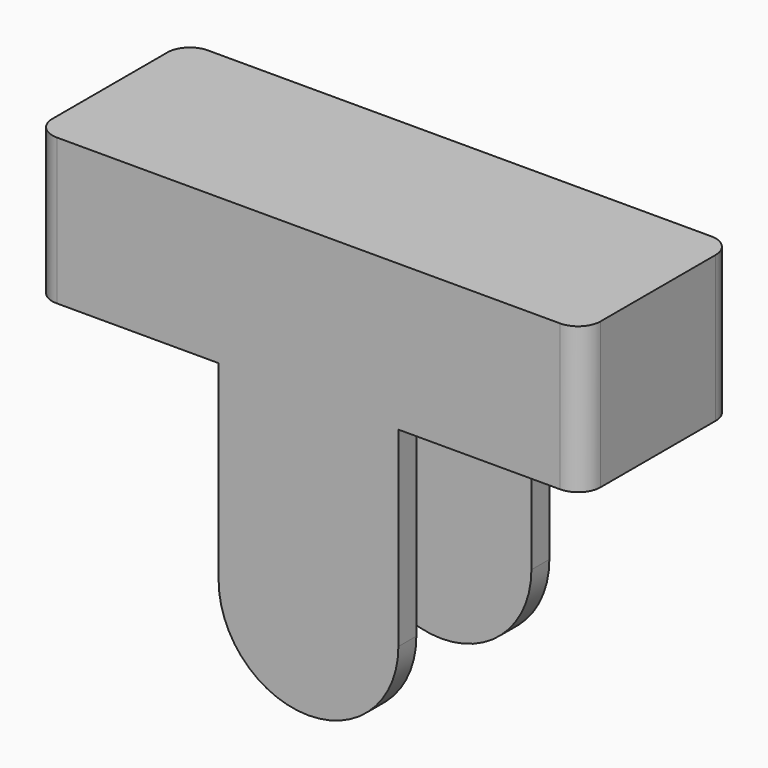
from build123d import *

# Parameters (mm, degrees)
F0_W     = 48.799998641
F0_H     = 16.799998641
F0_W_2   = 44.799998641
F0_H_2   = 12.799998641
F0_W_3   = 44
F0_H_3   = 12
F0_W_4   = 40
F0_H_4   = 8
F1_DEPTH = 13
F2_DEPTH = 10.5
F3_R     = 2
F4_R     = 2
F6_DEPTH = 25
F7_R     = 7.99999


# Not quite as in the source:
# - a fillet or chamfer is up to 0.001 mm smaller than in the source, because OpenCascade refuses the exact size


with BuildPart() as f1:
    # F0 (on Top) → F1 (new body)
    with BuildSketch(Plane.XY):
        Rectangle(F0_W, F0_H)
        Rectangle(F0_W_2, F0_H_2, mode=Mode.SUBTRACT)
        Rectangle(F0_W_2, F0_H_2)
        Rectangle(F0_W_3, F0_H_3, mode=Mode.SUBTRACT)
        Rectangle(F0_W_3, F0_H_3)
        Rectangle(F0_W_4, F0_H_4, mode=Mode.SUBTRACT)
        Rectangle(F0_W_4, F0_H_4)
    extrude(amount=F1_DEPTH)

    # F0 (on Top) → F2 (cut)
    with BuildSketch(Plane.XY):
        Rectangle(F0_W_2, F0_H_2)
        Rectangle(F0_W_3, F0_H_3, mode=Mode.SUBTRACT)
        Rectangle(F0_W_3, F0_H_3)
        Rectangle(F0_W_4, F0_H_4, mode=Mode.SUBTRACT)
        Rectangle(F0_W_4, F0_H_4)
    extrude(amount=F2_DEPTH, mode=Mode.SUBTRACT)

    # F3
    f3_edges = [f1.edges().sort_by_distance(p)[0] for p in [
        (-24.399999, -8.399999, 6.5),
        (-24.399999, 8.399999, 6.5),
        (24.399999, -8.399999, 6.5),
        (24.399999, 8.399999, 6.5),
    ]]
    fillet(f3_edges, radius=F3_R)

    # F4
    f4_edges = [f1.edges().sort_by_distance(p)[0] for p in [
        (-22.399999, -6.399999, 5.25),
        (22.399999, -6.399999, 5.25),
        (22.399999, 6.399999, 5.25),
        (-22.399999, 6.399999, 5.25),
    ]]
    fillet(f4_edges, radius=F4_R)

    # F5 (on face) → F6 (join)
    with BuildSketch(Plane(origin=(0, 0, 0), x_dir=(1, 0, 0), z_dir=(0, 0, -1))):
        Polygon((-8, 6.3999993205), (0, 6.3999993205), (8, 6.3999993205), (8, 8.3999993205), (-8, 8.3999993205), align=None)
        Polygon((8, -8.3999993205), (8, -6.3999993205), (0, -6.3999993205), (-8, -6.3999993205), (-8, -8.3999993205), align=None)
    extrude(amount=F6_DEPTH)

    # F7 (radius 8 in the source; OpenCascade refuses exactly that, so slightly less here)
    f7_edges = [f1.edges().sort_by_distance(p)[0] for p in [
        (-8, -7.399999, -25),
        (8, -7.399999, -25),
        (-8, 7.399999, -25),
        (8, 7.399999, -25),
    ]]
    fillet(f7_edges, radius=F7_R)


solid = f1.part
